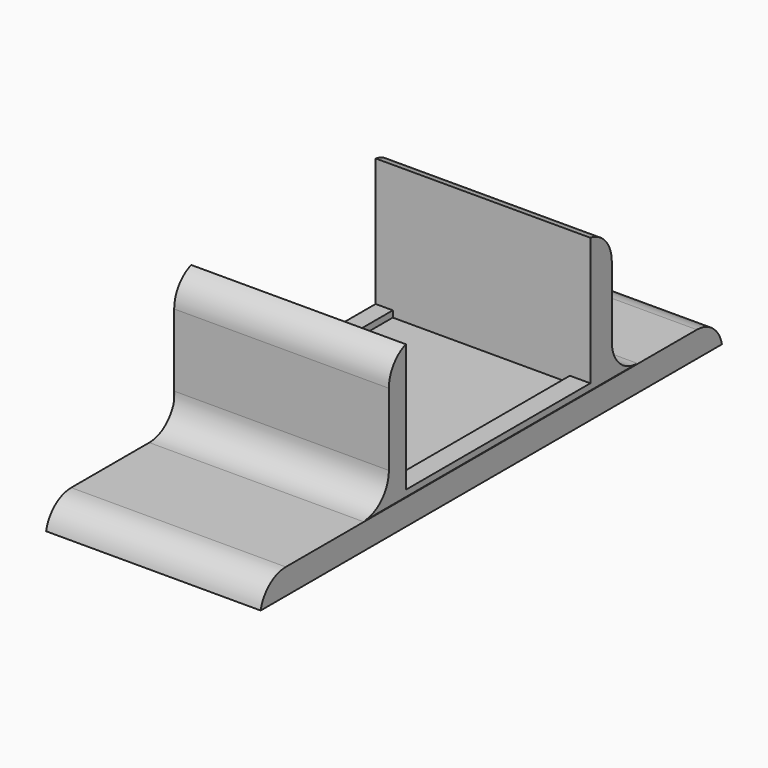
from build123d import *

# Parameters (mm, degrees)
F1_W        = 33.513052389
F1_H        = 43.4953216463
F2_DEPTH    = 25
F0_W        = 27.636364032
F0_H        = 36
F3_DEPTH    = 25
F4_W        = 33.513052389
F4_H        = 36
F5_DEPTH    = 20
F6_T1_DEPTH = 58.1822545614
F6_T3_DEPTH = 57.0345340949
F7_W        = 34
F7_H        = 90
F8_DEPTH    = 4
F9_T1_DEPTH = 58.4948974279
F10_R       = 5
F11_DEPTH   = 0.5


# Not quite as in the source:
# - a fillet or chamfer that OpenCascade refuses, or shapes differently, is made with other operations: its cross-section is extruded or revolved along the edge and cut away or added


with BuildPart() as f2:
    # F1 (on Top) → F2 (new body)
    with BuildSketch(Plane.XY):
        with Locations((-35.7246743515, 1.4273980632)):
            Rectangle(F1_W, F1_H)
    extrude(amount=F2_DEPTH)

    # F0 (on Top) → F3 (cut)
    with BuildSketch(Plane.XY):
        with Locations((-35.9798576683, 0.9857490659)):
            Rectangle(F0_W, F0_H)
    extrude(amount=F3_DEPTH, mode=Mode.SUBTRACT)

    # F4 (on face) → F5 (cut)
    with BuildSketch(Plane.XY.offset(25)):
        with Locations((-35.7246743515, 0.9857490659)):
            Rectangle(F4_W, F4_H)
    extrude(amount=-F5_DEPTH, mode=Mode.SUBTRACT)

    # F6: fillet of radius 5 on 2 edges, made by hand

    # F6_s2 → F6_t1 (cut)
    with BuildSketch(Plane.YZ.offset(-64.8158016322)):
        with BuildLine():
            ThreePointArc((23.1750588864, 20.0661595655), (21.9864530472, 23.302403461), (18.9857490659, 25))
            Line((18.9857490659, 25), (23.1750588864, 25))
            Line((23.1750588864, 25), (23.1750588864, 20.0661595655))
        make_face()
    extrude(amount=F6_T1_DEPTH, mode=Mode.SUBTRACT)

    # F6_s4 → F6_t3 (cut)
    with BuildSketch(Plane.YZ.offset(-64.241941399)):
        with BuildLine():
            ThreePointArc((-17.0142509341, 25), (-19.4111025802, 23.170600103), (-20.3202627599, 20.2957036588))
            Line((-20.3202627599, 20.2957036588), (-20.3202627599, 25))
            Line((-20.3202627599, 25), (-17.0142509341, 25))
        make_face()
    extrude(amount=F6_T3_DEPTH, mode=Mode.SUBTRACT)

    # F7 (on Top) → F8 (join)
    with BuildSketch(Plane.XY):
        with Locations((-35.3662480154, -0.4606725276)):
            Rectangle(F7_W, F7_H)
    extrude(amount=F8_DEPTH)

    # F9: fillet of radius 5 on 2 edges, made by hand

    # F9_s2 → F9_t1 (cut)
    with BuildSketch(Plane.YZ.offset(-64.6136967294)):
        with BuildLine():
            ThreePointArc((-40.561693042, 4), (-43.7239707021, 2.8729833462), (-45.4606725275, 0))
            Line((-45.4606725275, 0), (-45.4606725276, 4))
            Line((-45.4606725276, 4), (-40.561693042, 4))
        make_face()
        with BuildLine():
            ThreePointArc((39.6403479869, 4), (42.802625647, 2.8729833462), (44.5393274724, 0))
            Line((44.5393274724, 0), (44.5393274724, 4))
            Line((44.5393274724, 4), (39.6403479869, 4))
        make_face()
    extrude(amount=F9_T1_DEPTH, mode=Mode.SUBTRACT)

    # F10
    f10_edges = [f2.edges().sort_by_distance(p)[0] for p in [
        (-35.667198, -20.320263, 4),
        (-35.667198, 23.175059, 4),
    ]]
    fillet(f10_edges, radius=F10_R)

    # F11 (cut): a face of the model
    f11_faces = [f2.faces().sort_by_distance(p)[0] for p in [
        (-18.3662480154, -0.4606725276, 1.9725049158),
    ]]
    extrude(f11_faces, amount=-F11_DEPTH, mode=Mode.SUBTRACT)


solid = f2.part
